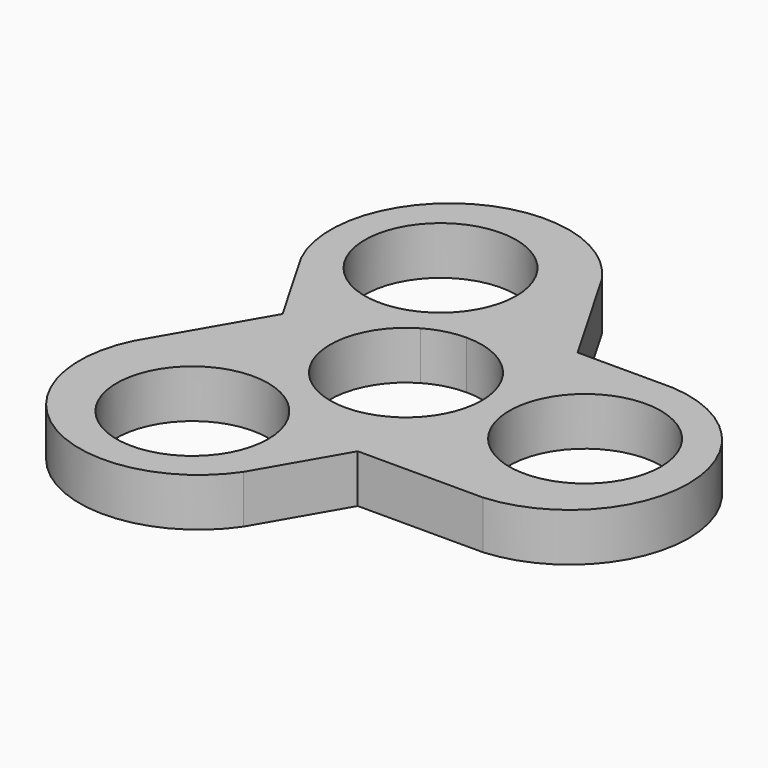
from build123d import *

# Parameters (mm, degrees)
F0_R            = 11
F1_DEPTH        = 7
F1_COPIES_COUNT = 3


# Not quite as in the source:
# - a pattern or mirror of a feature is missing from the dataset's text; its kind, count and spacing are read off the source's solid


with BuildPart() as f1:
    # F0 (on Top) → F1 (new body)
    with BuildSketch(Plane.XY):
        with BuildLine():
            ThreePointArc((0, 11), (7.7781745931, 7.7781745931), (11, 0))
            ThreePointArc((11, 0), (7.7781745931, -7.7781745931), (0, -11))
            Line((0, -11), (0, -18.5))
            Line((0, -18.5), (26, -18.5))
            ThreePointArc((26, -18.5), (42.0452305564, -1.25), (26, 16))
            Line((26, 16), (0, 16))
            Line((0, 16), (0, 11))
        make_face()
        with Locations((26, 0)):
            Circle(F0_R, mode=Mode.SUBTRACT)
    extrude(amount=F1_DEPTH)

    # F1_copies: F1 ×3 about axis
    f1_copies_axis = Axis((0, 0, 0), (0, 0, 1))


with BuildPart() as f1_1:
    add(f1.part)
    for i in range(1, F1_COPIES_COUNT):
        add(f1.part.rotate(f1_copies_axis, i * 360 / F1_COPIES_COUNT))


solid = f1_1.part
